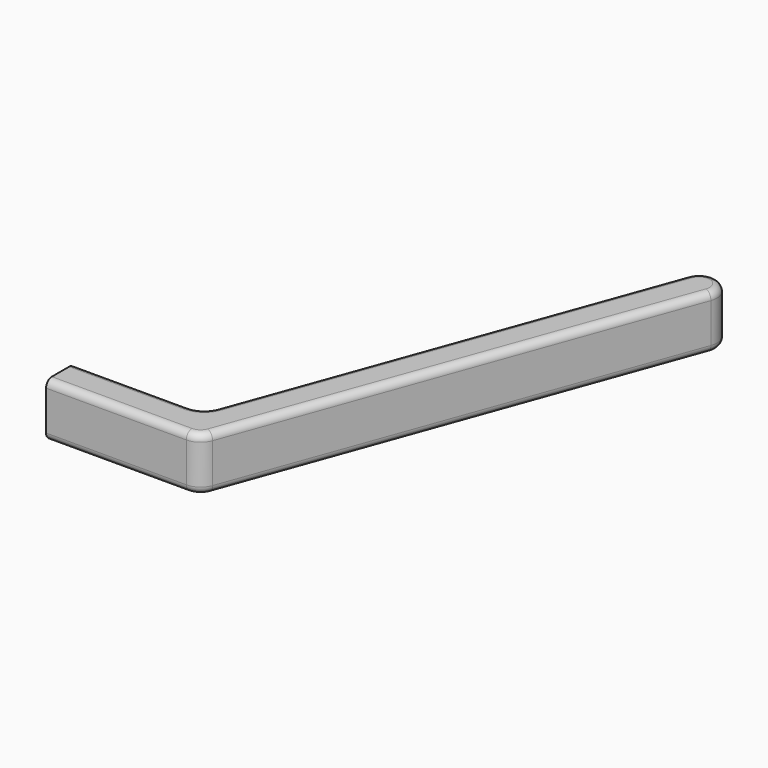
from build123d import *

# Parameters (mm, degrees)
F1_DEPTH = 15
F2_R     = 4.99999
F3_R     = 2


# Not quite as in the source:
# - a fillet or chamfer is up to 0.001 mm smaller than in the source, because OpenCascade refuses the exact size


with BuildPart() as f1:
    # F0 (on Top) → F1 (new body)
    with BuildSketch(Plane.XY):
        Polygon((0, 10), (0, 0), (42.567110899, 0), (88.8907263303, 127.2730873849), (79.4938001224, 130.6932888181), (35.5650355169, 10), align=None)
    extrude(amount=F1_DEPTH)

    # F2 (radius 5 in the source; OpenCascade refuses exactly that, so slightly less here)
    f2_edges = [f1.edges().sort_by_distance(p)[0] for p in [
        (35.565036, 10, 7.5),
        (42.567111, 0, 7.5),
        (79.4938, 130.693289, 7.5),
        (88.890726, 127.273087, 7.5),
    ]]
    fillet(f2_edges, radius=F2_R)

    # F3
    f3_edges = [f1.edges().sort_by_distance(p)[0] for p in [
        (57.273081, 69.642364, 15),
        (57.273081, 69.642364, 0),
    ]]
    fillet(f3_edges, radius=F3_R)


solid = f1.part
